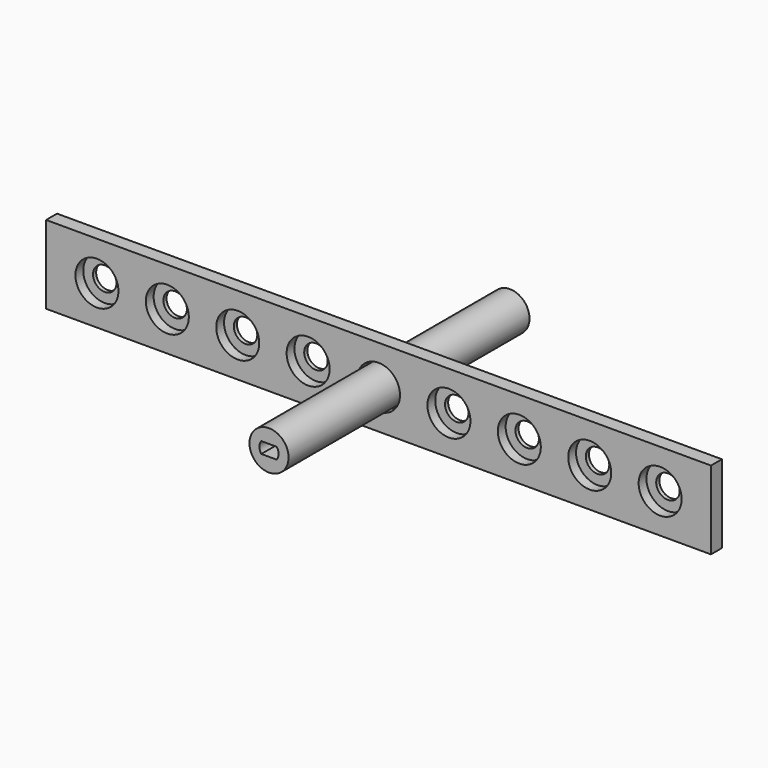
from build123d import *

# Parameters (mm, degrees)
F0_R     = 5
F1_DEPTH = 38.5
F2_W     = 170
F2_H     = 20
F2_R     = 5.5
F3_DEPTH = 3.5
F2_R_2   = 3
F4_DEPTH = 1


with BuildPart() as f1:
    # F0 (on Front) → F1 (new body, symmetric)
    with BuildSketch(Plane.XZ):
        Circle(F0_R)
        with BuildLine():
            ThreePointArc((-1.9748417658, -1.45), (-2.45, 0), (-1.9748417658, 1.45))
            Line((-1.9748417658, 1.45), (1.9748417658, 1.45))
            ThreePointArc((1.9748417658, 1.45), (2.45, 0), (1.9748417658, -1.45))
            Line((1.9748417658, -1.45), (-1.9748417658, -1.45))
        make_face(mode=Mode.SUBTRACT)
    extrude(amount=F1_DEPTH, both=True)


with BuildPart() as f3:
    # F2 (on Front) → F3 (new body)
    with BuildSketch(Plane.XZ):
        Rectangle(F2_W, F2_H)
        with Locations((-72, 0)):
            Circle(F2_R, mode=Mode.SUBTRACT)
        with Locations((-54, 0)):
            Circle(F2_R, mode=Mode.SUBTRACT)
        with Locations((-36, 0)):
            Circle(F2_R, mode=Mode.SUBTRACT)
        with Locations((-18, 0)):
            Circle(F2_R, mode=Mode.SUBTRACT)
        Circle(F2_R, mode=Mode.SUBTRACT)
        with Locations((18, 0)):
            Circle(F2_R, mode=Mode.SUBTRACT)
        with Locations((36, 0)):
            Circle(F2_R, mode=Mode.SUBTRACT)
        with Locations((54, 0)):
            Circle(F2_R, mode=Mode.SUBTRACT)
        with Locations((72, 0)):
            Circle(F2_R, mode=Mode.SUBTRACT)
    extrude(amount=F3_DEPTH)

    # F2 (on Front) → F4 (join)
    with BuildSketch(Plane.XZ):
        with Locations((-72, 0)):
            Circle(F2_R)
        with Locations((-72, 0)):
            Circle(F2_R_2, mode=Mode.SUBTRACT)
        with Locations((-54, 0)):
            Circle(F2_R)
        with Locations((-54, 0)):
            Circle(F2_R_2, mode=Mode.SUBTRACT)
        with Locations((-36, 0)):
            Circle(F2_R)
        with Locations((-36, 0)):
            Circle(F2_R_2, mode=Mode.SUBTRACT)
        with Locations((-18, 0)):
            Circle(F2_R)
        with Locations((-18, 0)):
            Circle(F2_R_2, mode=Mode.SUBTRACT)
        Circle(F2_R)
        Circle(F2_R_2, mode=Mode.SUBTRACT)
        with Locations((18, 0)):
            Circle(F2_R)
        with Locations((18, 0)):
            Circle(F2_R_2, mode=Mode.SUBTRACT)
        with Locations((36, 0)):
            Circle(F2_R)
        with Locations((36, 0)):
            Circle(F2_R_2, mode=Mode.SUBTRACT)
        with Locations((54, 0)):
            Circle(F2_R)
        with Locations((54, 0)):
            Circle(F2_R_2, mode=Mode.SUBTRACT)
        with Locations((72, 0)):
            Circle(F2_R)
        with Locations((72, 0)):
            Circle(F2_R_2, mode=Mode.SUBTRACT)
    extrude(amount=F4_DEPTH)


solid = Compound([f1.part, f3.part])
